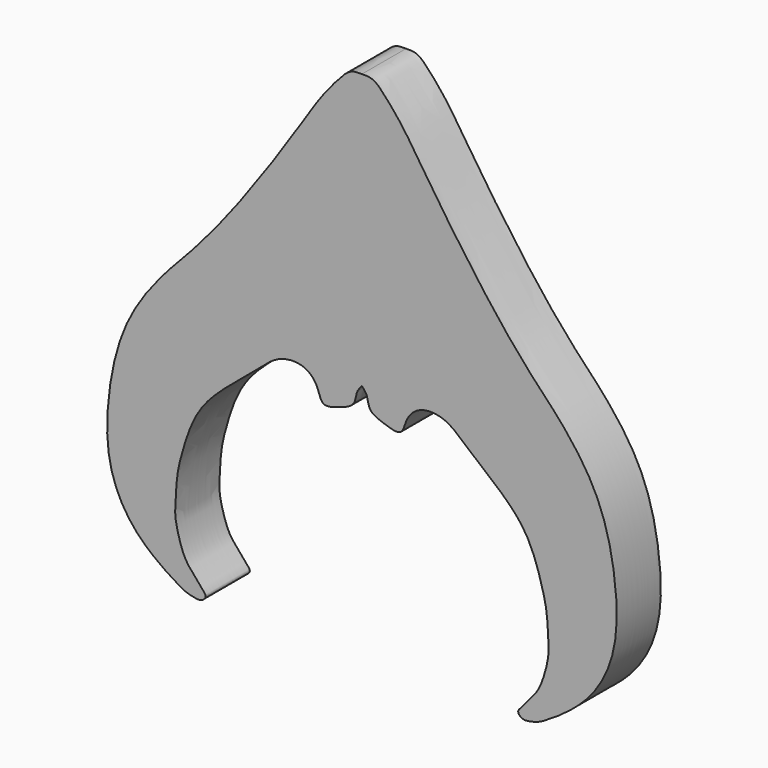
from build123d import *

# Parameters (mm, degrees)
F2_DEPTH = 4


# Not quite as in the source:
# - the dataset's text gives a spline's control points without its knots; the knots are read off the source's solid


with BuildPart() as f2:
    # F0 (on Front) → F2 (new body)
    with BuildSketch(Plane.XZ):
        with BuildLine():
            add(Edge.make_bspline(
                [(0, 18.694814), (0.281487, 18.699279), (0.865345, 18.708539), (3.30752, 16.10989), (3.702386, 14.972987), (8.73213, 7.769785), (11.155721, 4.614056), (14.693458, 0.959631), (17.308111, -2.393977), (18.495282, -7.508713), (18.576512, -12.235854), (16.659146, -15.96978), (13.908616, -17.896495), (12.630329, -18.61843), (11.624836, -18.727539), (11.222412, -18.380298), (11.762197, -17.616961), (12.714426, -16.82937), (13.646661, -14.126365), (13.501646, -13.294972), (13.454721, -11.301442), (13.109164, -9.909659), (12.18093, -6.763611), (9.933007, -4.487593), (7.80721, -2.882594), (6.102385, -1.229456), (4.147432, -1.137568), (3.187214, -2.181197), (2.928591, -3.529645), (1.575755, -3.076182), (0.448772, -2.695916), (0.434155, -1.696179), (0.126912, -1.35555), (0, -1.214847)],
                knots=[0, 0, 0, 0, 0.011913, 0.02471, 0.116497, 0.13487, 0.190071, 0.201025, 0.237509, 0.273562, 0.30515, 0.330285, 0.356059, 0.366119, 0.367638, 0.370849, 0.372702, 0.384317, 0.388696, 0.412113, 0.423174, 0.496377, 0.584711, 0.659351, 0.744255, 0.794728, 0.84155, 0.877412, 0.900586, 0.930508, 0.965365, 0.985693, 1, 1, 1, 1], degree=3))
            add(Edge.make_bspline(
                [(0, 18.694814), (-0.281488, 18.699279), (-0.865345, 18.708539), (-3.30752, 16.10989), (-3.702386, 14.972987), (-8.73213, 7.769785), (-11.155722, 4.614056), (-14.693458, 0.959631), (-17.308111, -2.393977), (-18.495282, -7.508713), (-18.576512, -12.235854), (-16.659146, -15.96978), (-13.908616, -17.896495), (-12.630329, -18.61843), (-11.624836, -18.727539), (-11.222412, -18.380298), (-11.762197, -17.616961), (-12.714426, -16.82937), (-13.646661, -14.126365), (-13.501646, -13.294972), (-13.454721, -11.301442), (-13.109164, -9.909659), (-12.18093, -6.763611), (-9.933008, -4.487593), (-7.807211, -2.882594), (-6.102386, -1.229456), (-4.147432, -1.137568), (-3.187214, -2.181197), (-2.928591, -3.529645), (-1.575755, -3.076182), (-0.448773, -2.695916), (-0.434155, -1.696179), (-0.126912, -1.35555), (0, -1.214847)],
                knots=[0, 0, 0, 0, 0.011913, 0.02471, 0.116497, 0.13487, 0.190071, 0.201025, 0.237509, 0.273562, 0.30515, 0.330285, 0.356059, 0.366119, 0.367638, 0.370849, 0.372702, 0.384317, 0.388696, 0.412113, 0.423174, 0.496377, 0.584711, 0.659351, 0.744255, 0.794728, 0.84155, 0.877412, 0.900586, 0.930508, 0.965365, 0.985693, 1, 1, 1, 1], degree=3))
        make_face()
    extrude(amount=F2_DEPTH)


solid = f2.part
